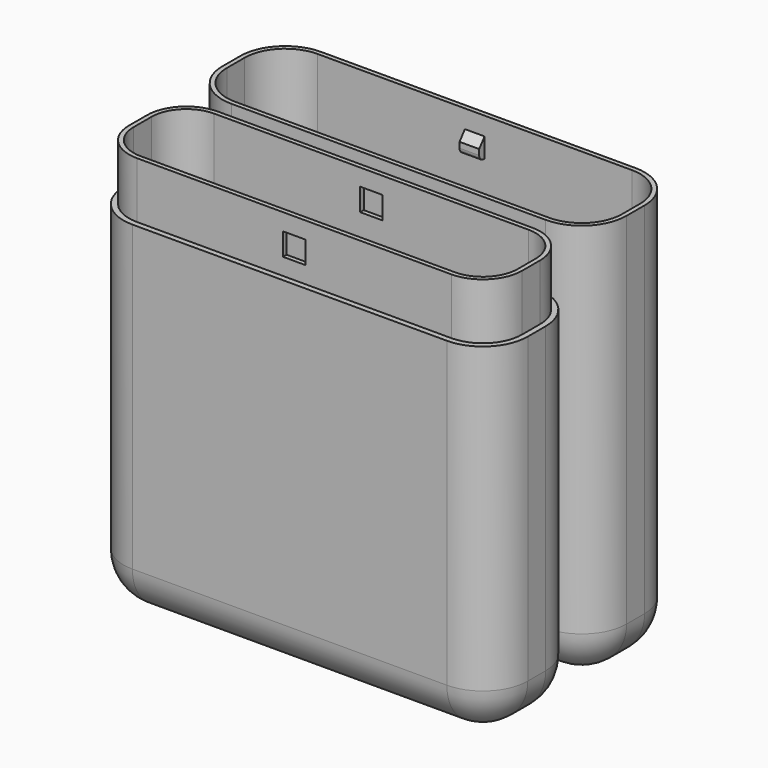
from build123d import *

# Parameters (mm, degrees)
F0_W      = 72
F0_H      = 20
F1_DEPTH  = 72
F2_R      = 8
F2_2_R    = 8
F3_T      = -0.8
F3_2_T    = -0.8
F4_W      = 3.5
F4_H      = 3.5
F5_DEPTH  = 1.2
F6_R      = 1
F7_SIZE2  = 1.49999
F7_SIZE   = 1.19999
F10_DEPTH = 10
F12_DEPTH = 3
F14_DEPTH = 10
F15_W     = 4
F15_H     = 4
F16_DEPTH = 25
F17_SIZE  = 0.99999


# Not quite as in the source:
# - a fillet or chamfer is up to 0.001 mm smaller than in the source, because OpenCascade refuses the exact size


with BuildPart() as f1:
    # F0 (on Top) → F1 (new body)
    with BuildSketch(Plane.XY):
        with Locations((36, 10)):
            Rectangle(F0_W, F0_H)
    extrude(amount=F1_DEPTH)

    # F2
    f2_edges = [f1.edges().sort_by_distance(p)[0] for p in [
        (0, 20, 36),
        (0, 0, 36),
        (0, 10, 0),
        (36, 20, 0),
        (36, 0, 0),
        (72, 20, 36),
        (72, 10, 0),
        (72, 0, 36),
    ]]
    fillet(f2_edges, radius=F2_R)

    # F3
    f3_openings = [f1.faces().sort_by_distance(p)[0] for p in [
        (36, 10, 72),
    ]]
    offset(amount=F3_T, openings=f3_openings)

    # F4 (on face) → F5 (join)
    with BuildSketch(Plane(origin=(0, 0.8, 0), x_dir=(-1, 0, 0), z_dir=(0, 1, 0))):
        with Locations((-36, 67)):
            Rectangle(F4_W, F4_H)
    extrude(amount=F5_DEPTH)

    # F6
    f6_edges = [f1.edges().sort_by_distance(p)[0] for p in [
        (36, 2, 65.25),
    ]]
    fillet(f6_edges, radius=F6_R)

    # F7 (size 1.2 and 1.5 in the source; OpenCascade refuses exactly that, so slightly less here)
    f7_edges = [f1.edges().sort_by_distance(p)[0] for p in [
        (36, 2, 68.75),
    ]]
    f7_side = f1.faces().sort_by_distance((36, 1.4, 68.75))[0]
    chamfer(f7_edges, length=F7_SIZE, length2=F7_SIZE2, reference=f7_side)

    # F9: F1 across plane


with BuildPart() as f1b:
    # F0 (on Top) → F1, piece 2 (new body)
    with BuildSketch(Plane.XY):
        with Locations((36, -12)):
            Rectangle(F0_W, F0_H)
    extrude(amount=F1_DEPTH)

    # F2#2
    f2_2_edges = [f1b.edges().sort_by_distance(p)[0] for p in [
        (0, -2, 36),
        (0, -22, 36),
        (72, -22, 36),
        (72, -2, 36),
        (72, -12, 0),
        (36, -2, 0),
        (36, -22, 0),
        (0, -12, 0),
    ]]
    fillet(f2_2_edges, radius=F2_2_R)

    # F3#2
    f3_2_openings = [f1b.faces().sort_by_distance(p)[0] for p in [
        (36, -12, 72),
    ]]
    offset(amount=F3_2_T, openings=f3_2_openings)

    # F10 (cut): a face of the model
    f10_faces = [f1b.faces().sort_by_distance(p)[0] for p in [
        (36, -2.7472616677, 72),
    ]]
    extrude(f10_faces, amount=-F10_DEPTH, mode=Mode.SUBTRACT)

    # F11 (on face) → F12 (join)
    with BuildSketch(Plane.XY.offset(62)):
        with BuildLine():
            ThreePointArc((72, -10), (69.6568542495, -4.3431457505), (64, -2))
            Line((64, -2), (8, -2))
            ThreePointArc((8, -2), (2.3431457505, -4.3431457505), (0, -10))
            Line((0, -10), (0, -14))
            ThreePointArc((0, -14), (2.3431457505, -19.6568542495), (8, -22))
            Line((8, -22), (64, -22))
            ThreePointArc((64, -22), (69.6568542495, -19.6568542495), (72, -14))
            Line((72, -14), (72, -10))
        make_face()
        with BuildLine():
            ThreePointArc((0.8, -10), (2.9088311755, -4.9088311755), (8, -2.8))
            Line((8, -2.8), (64, -2.8))
            ThreePointArc((64, -2.8), (69.0911688245, -4.9088311755), (71.2, -10))
            Line((71.2, -10), (71.2, -14))
            ThreePointArc((71.2, -14), (69.0911688245, -19.0911688245), (64, -21.2))
            Line((64, -21.2), (8, -21.2))
            ThreePointArc((8, -21.2), (2.9088311755, -19.0911688245), (0.8, -14))
            Line((0.8, -14), (0.8, -10))
        make_face(mode=Mode.SUBTRACT)
        with BuildLine():
            Line((64, -2.8), (8, -2.8))
            ThreePointArc((8, -2.8), (2.9088311755, -4.9088311755), (0.8, -10))
            Line((0.8, -10), (0.8, -14))
            ThreePointArc((0.8, -14), (2.9088311755, -19.0911688245), (8, -21.2))
            Line((8, -21.2), (64, -21.2))
            ThreePointArc((64, -21.2), (69.0911688245, -19.0911688245), (71.2, -14))
            Line((71.2, -14), (71.2, -10))
            ThreePointArc((71.2, -10), (69.0911688245, -4.9088311755), (64, -2.8))
        make_face()
        with BuildLine():
            ThreePointArc((1.8, -10), (3.6159379566, -5.6159379566), (8, -3.8))
            Line((8, -3.8), (64, -3.8))
            ThreePointArc((64, -3.8), (68.3840620434, -5.6159379566), (70.2, -10))
            Line((70.2, -10), (70.2, -14))
            ThreePointArc((70.2, -14), (68.3840620434, -18.3840620434), (64, -20.2))
            Line((64, -20.2), (8, -20.2))
            ThreePointArc((8, -20.2), (3.6159379566, -18.3840620434), (1.8, -14))
            Line((1.8, -14), (1.8, -10))
        make_face(mode=Mode.SUBTRACT)
    extrude(amount=-F12_DEPTH)

    # F13 (on face) → F14 (join)
    with BuildSketch(Plane.XY.offset(62)):
        with BuildLine():
            Line((64, -3), (8, -3))
            ThreePointArc((8, -3), (3.0502525317, -5.0502525317), (1, -10))
            Line((1, -10), (1, -14))
            ThreePointArc((1, -14), (3.0502525317, -18.9497474683), (8, -21))
            Line((8, -21), (64, -21))
            ThreePointArc((64, -21), (68.9497474683, -18.9497474683), (71, -14))
            Line((71, -14), (71, -10))
            ThreePointArc((71, -10), (68.9497474683, -5.0502525317), (64, -3))
        make_face()
        with BuildLine():
            ThreePointArc((1.8, -10), (3.6159379566, -5.6159379566), (8, -3.8))
            Line((8, -3.8), (64, -3.8))
            ThreePointArc((64, -3.8), (68.3840620434, -5.6159379566), (70.2, -10))
            Line((70.2, -10), (70.2, -14))
            ThreePointArc((70.2, -14), (68.3840620434, -18.3840620434), (64, -20.2))
            Line((64, -20.2), (8, -20.2))
            ThreePointArc((8, -20.2), (3.6159379566, -18.3840620434), (1.8, -14))
            Line((1.8, -14), (1.8, -10))
        make_face(mode=Mode.SUBTRACT)
    extrude(amount=F14_DEPTH)

    # F15 (on face) → F16 (cut)
    with BuildSketch(Plane(origin=(0, -3, 0), x_dir=(-1, 0, 0), z_dir=(0, 1, 0))):
        with Locations((-36, 67)):
            Rectangle(F15_W, F15_H)
    extrude(amount=-F16_DEPTH, mode=Mode.SUBTRACT)

    # F17 (size 1 in the source; OpenCascade refuses exactly that, so slightly less here)
    f17_edges = [f1b.edges().sort_by_distance(p)[0] for p in [
        (36, -20.2, 59),
    ]]
    chamfer(f17_edges, length=F17_SIZE)


with BuildPart() as f1_1:
    add(f1.part)
    add(f1.part.mirror(Plane(origin=(36, 10, 39.9536991671), x_dir=(1, 0, 0), z_dir=(0, -1, 0))))


solid = Compound([f1b.part, f1_1.part])
